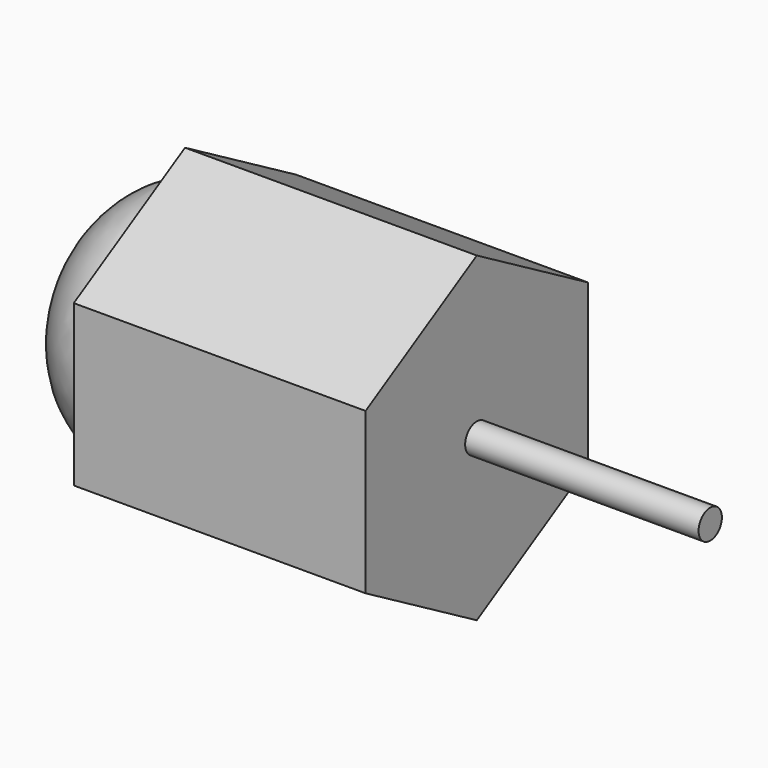
from build123d import *

# Parameters (mm, degrees)
F1_DEPTH     = 100
F2_R         = 5
F3_DEPTH     = 80
F6_TEXT_SIZE = 20.5364888196
F7_DEPTH     = 2.54
F8_TEXT_SIZE = 20.5641998735
F9_DEPTH     = 5


# Not quite as in the source:
# - Text() gives the source's letters only with a copy of the font that has no kerning and outlines rounded to 1/6400 em; it was checked with that copy


with BuildPart() as f1:
    # F0 (on Right) → F1 (new body)
    with BuildSketch(Plane.YZ):
        Polygon((47.6522482932, -27.5120383795), (47.6522482932, 27.5120383795), (0, 55.0240767591), (-47.6522482932, 27.5120383795), (-47.6522482932, -27.5120383795), (0, -55.0240767591), align=None)
    extrude(amount=F1_DEPTH)

    # F2 (on face) → F3 (join)
    with BuildSketch(Plane.YZ.offset(100)):
        Circle(F2_R)
    extrude(amount=F3_DEPTH)

    # F4 (on Front) → F5 (revolve)
    with BuildSketch(Plane.XZ):
        with BuildLine():
            Line((0, 0), (0, 41.966388))
            add(Edge.make_bspline(
                [(0, 41.966388), (-30.2231726094, 41.966388), (-33.5897337471, 4.6746386542)],
                knots=[3.1415926536, 3.1415926536, 3.1415926536, 4.6007672705, 4.6007672705, 4.6007672705], degree=2, weights=[1, 0.7454495503, 1]))
            ThreePointArc((-33.5897337471, 4.6746386542), (-37.0336694578, 3.3823644174), (-38.479448428, 0))
            Line((-38.479448428, 0), (0, 0))
        make_face()
    revolve(axis=Axis((-27.5958828417, 0, 0), (-1, 0, 0)))

    # F6 (on face) → F7 (join)
    with BuildSketch(Plane(origin=(0, 47.6522482932, 0), x_dir=(-1, 0, 0), z_dir=(0, 1, 0))):
        with Locations((-86.7541972705, 5.2555497708)):
            Text('TOMA 2', F6_TEXT_SIZE, font='Open Sans', text_align=(TextAlign.LEFT, TextAlign.BOTTOM))
    extrude(amount=F7_DEPTH)

    # F8 (on face) → F9 (cut)
    with BuildSketch(Plane(origin=(0, 23.8261241466, -41.2680575693), x_dir=(1, 0, 0), z_dir=(0, 0.5, -0.8660254038))):
        with Locations((12.3490262243, -7.1114962017)):
            Text('TOMA 3', F8_TEXT_SIZE, font='Open Sans', text_align=(TextAlign.LEFT, TextAlign.BOTTOM))
    extrude(amount=-F9_DEPTH, mode=Mode.SUBTRACT)


solid = f1.part
